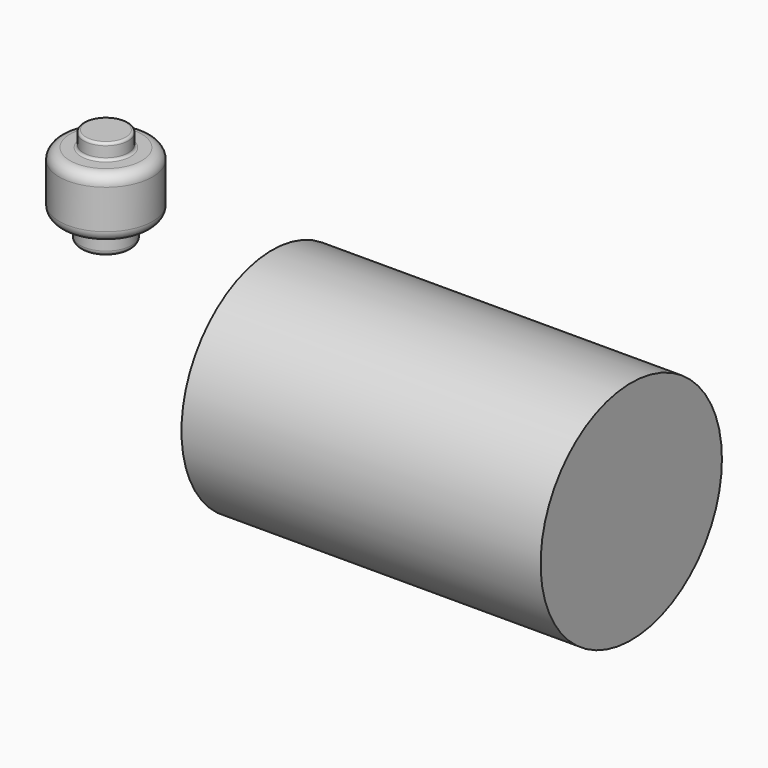
from build123d import *

# Parameters (mm, degrees)
F2_R     = 2.145498841
F4_R     = 0.4903403449
F6_D     = 6.35
F6_DEPTH = 6.35
F6_TIP   = 1.9077324654
F7_R     = 1.0187545891
F3_R     = 22.4683237684
F8_DEPTH = 71.223795414


with BuildPart() as f1:
    # F0 (on Front) → F1 (revolve)
    with BuildSketch(Plane.XZ):
        Polygon((4.4335573912, 19.5186324418), (0, 19.5186324418), (0, 0), (5.1236599684, 0), (5.1236599684, 4.3991170824), (9.2642754316, 4.3991170824), (9.2642754316, 16.4445396513), (4.4335573912, 16.4445396513), align=None)
    revolve(axis=Axis((0, 0, 9.7593162209), (0, 0, 1)))

    # F2
    f2_edges = [f1.edges().sort_by_distance(p)[0] for p in [
        (-9.264275, 0, 16.44454),
        (-9.264275, 0, 4.399117),
        (9.264275, 0, 10.421828),
    ]]
    fillet(f2_edges, radius=F2_R)

    # F4
    f4_edges = [f1.edges().sort_by_distance(p)[0] for p in [
        (-4.433557, 0, 19.518632),
        (-4.433557, 0, 16.44454),
        (4.433557, 0, 17.981586),
    ]]
    fillet(f4_edges, radius=F4_R)

    # F6
    with Locations(Plane(origin=(0, 0, 0), x_dir=(1, 0, 0), z_dir=(0, 0, -1))):
        with Locations((0, 0)):
            Hole(F6_D / 2, depth=F6_DEPTH)
            with Locations((0, 0, -(F6_DEPTH + F6_TIP / 2))):  # 118° drill point
                Cone(0, F6_D / 2, F6_TIP, mode=Mode.SUBTRACT)

    # F7
    f7_edges = [f1.edges().sort_by_distance(p)[0] for p in [
        (-9.264275, 0, 6.544616),
        (-5.12366, 0, 0),
        (-9.264275, 0, 14.299041),
        (-4.433557, 0, 19.028292),
    ]]
    fillet(f7_edges, radius=F7_R)


with BuildPart() as f8:
    # F3 (on Right) → F8 (new body)
    with BuildSketch(Plane.YZ):
        with Locations((41.1928445101, -40.6823679805)):
            Circle(F3_R)
    extrude(amount=F8_DEPTH)


solid = Compound([f1.part, f8.part])
